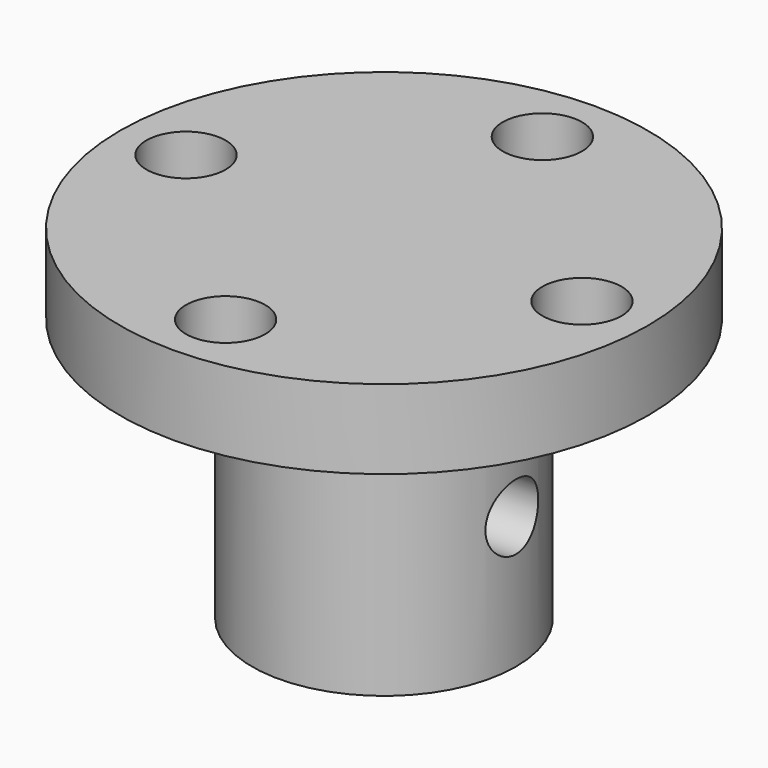
from build123d import *

# Parameters (mm, degrees)
F0_R     = 5
F1_DEPTH = 10
F2_R     = 1.25
F3_DEPTH = 3.5
F4_R     = 10
F4_R_2   = 1.5
F4_R_3   = 5
F5_DEPTH = 3


with BuildPart() as f1:
    # F0 (on Top) → F1 (new body)
    with BuildSketch(Plane.XY):
        Circle(F0_R)
        with BuildLine():
            ThreePointArc((1.5, 2), (2.2360679775, 1.1180339887), (2.5, 0))
            ThreePointArc((2.5, 0), (2.2360679775, -1.1180339887), (1.5, -2))
            ThreePointArc((1.5, -2), (-2.5, 0), (1.5, 2))
        make_face(mode=Mode.SUBTRACT)
        with BuildLine():
            ThreePointArc((1.5, -2), (2.2360679775, -1.1180339887), (2.5, 0))
            ThreePointArc((2.5, 0), (2.2360679775, 1.1180339887), (1.5, 2))
            Line((1.5, 2), (1.5, -2))
        make_face()
    extrude(amount=F1_DEPTH)

    # F2 (on face) → F3 (cut, through all)
    with BuildSketch(Plane(origin=(1.5, 0, 0), x_dir=(0, -1, 0), z_dir=(-1, 0, 0))):
        with Locations((0, 5)):
            Circle(F2_R)
    extrude(amount=-F3_DEPTH, mode=Mode.SUBTRACT)

    # F4 (on face) → F5 (join)
    with BuildSketch(Plane.XY.offset(10)):
        Circle(F4_R)
        with Locations((0, -7.5)):
            Circle(F4_R_2, mode=Mode.SUBTRACT)
        with Locations((-7.5, 0)):
            Circle(F4_R_2, mode=Mode.SUBTRACT)
        Circle(F4_R_3, mode=Mode.SUBTRACT)
        with Locations((7.5, 0)):
            Circle(F4_R_2, mode=Mode.SUBTRACT)
        with Locations((0, 7.5)):
            Circle(F4_R_2, mode=Mode.SUBTRACT)
        Circle(F4_R_3)
        with BuildLine():
            Line((1.5, 2), (1.5, -2))
            ThreePointArc((1.5, -2), (-2.5, 0), (1.5, 2))
        make_face(mode=Mode.SUBTRACT)
        with BuildLine():
            ThreePointArc((1.5, 2), (-2.5, 0), (1.5, -2))
            Line((1.5, -2), (1.5, 2))
        make_face()
    extrude(amount=F5_DEPTH)


solid = f1.part
